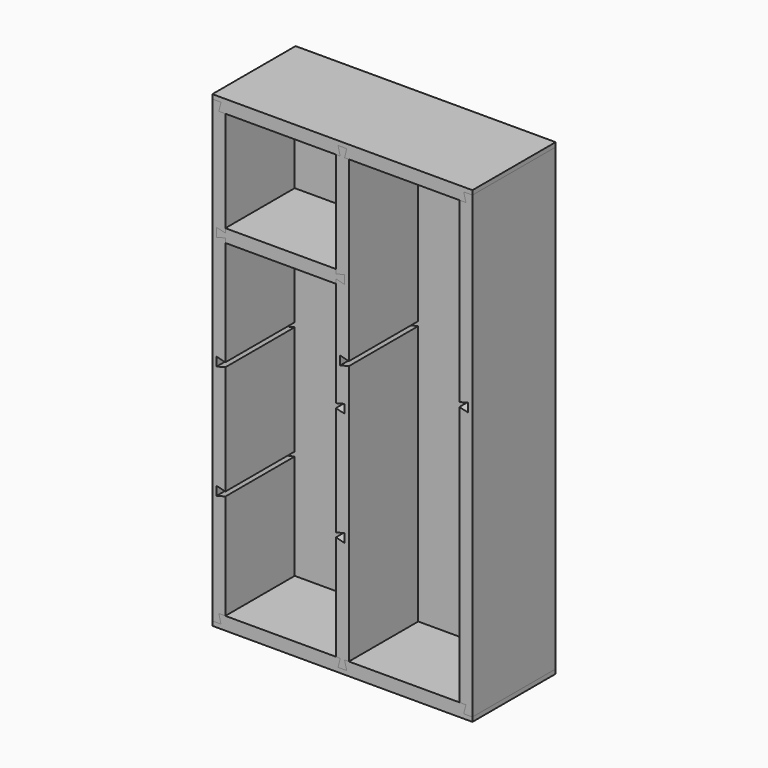
from build123d import *

# Parameters (mm, degrees)
F1_DEPTH  = 152.4
F2_DEPTH  = 152.4
F3_W      = 19.05
F3_H      = 19.05
F4_DEPTH  = 12.7
F6_W      = 361.95
F6_H      = 666.75
F7_DEPTH  = 5.55625
F8_W      = 360.3625
F8_H      = 665.1625
F9_DEPTH  = 4.99999
F11_DEPTH = 127
F13_DEPTH = 127


# Not quite as in the source:
# - a feature names something its author has since deleted; it is built from what else it names


with BuildPart() as f1:
    # F0 (on Front) → F1 (new body)
    with BuildSketch(Plane.XZ):
        Polygon((-180.9664656361, 323.85), (-190.5, 323.85), (-190.5, -323.85), (-180.9664656361, -323.85), (-171.45, -323.85), (-171.45, -176.2125), (-171.45, -169.8710343639), (-184.15, -173.0375), (-184.15, -160.3375), (-171.45, -163.5039656361), (-171.45, -157.1625), (-171.45, -9.525), (-171.45, -3.1835343639), (-184.15, -6.35), (-184.15, 6.35), (-171.45, 3.1835343639), (-171.45, 9.525), (-171.45, 157.1625), (-171.45, 163.5039656361), (-184.15, 160.3375), (-184.15, 173.0375), (-171.45, 169.8710343639), (-171.45, 176.2125), (-171.45, 323.85), align=None)
        Polygon((-177.8, 336.55), (-190.5, 336.55), (-190.5, 323.85), (-180.9664656361, 323.85), align=None)
        Polygon((-180.9664656361, -323.85), (-190.5, -323.85), (-190.5, -336.55), (-177.8, -336.55), align=None)
    extrude(amount=F1_DEPTH)


with BuildPart() as f1b:
    # F0 (on Front) → F1, piece 2 (new body)
    with BuildSketch(Plane.XZ):
        Polygon((190.5, -323.85), (190.5, 323.85), (180.9664656361, 323.85), (171.45, 323.85), (171.45, 69.85), (171.45, 63.5085343639), (184.15, 66.675), (184.15, 53.975), (171.45, 57.1414656361), (171.45, 50.8), (171.45, -323.85), (180.9664656361, -323.85), align=None)
        Polygon((190.5, -336.55), (190.5, -323.85), (180.9664656361, -323.85), (177.8, -336.55), align=None)
        Polygon((190.5, 323.85), (190.5, 336.55), (177.8, 336.55), (180.9664656361, 323.85), align=None)
    extrude(amount=F1_DEPTH)


with BuildPart() as f2:
    # F0 (on Front) → F2 (new body, through all)
    with BuildSketch(Plane.XZ):
        Polygon((190.5, 336.55), (190.5, 342.9), (-190.5, 342.9), (-190.5, 336.55), (-177.8, 336.55), (-180.9664656361, 323.85), (-171.45, 323.85), (-9.525, 323.85), (-3.1835343639, 323.85), (-6.35, 336.55), (6.35, 336.55), (3.1835343639, 323.85), (9.525, 323.85), (171.45, 323.85), (180.9664656361, 323.85), (177.8, 336.55), align=None)
    extrude(amount=F2_DEPTH)


with BuildPart() as f2b:
    # F0 (on Front) → F2, piece 2 (new body, through all)
    with BuildSketch(Plane.XZ):
        Polygon((190.5, -342.9), (190.5, -336.55), (177.8, -336.55), (180.9664656361, -323.85), (171.45, -323.85), (9.525, -323.85), (9.525, -342.9), align=None)
        Polygon((-9.525, -342.9), (9.525, -342.9), (9.525, -323.85), (3.1835343639, -323.85), (6.35, -336.55), (-6.35, -336.55), (-3.1835343639, -323.85), (-9.525, -323.85), align=None)
        Polygon((-177.8, -336.55), (-190.5, -336.55), (-190.5, -342.9), (-9.525, -342.9), (-9.525, -323.85), (-171.45, -323.85), (-180.9664656361, -323.85), align=None)
    extrude(amount=F2_DEPTH)

    # F3 (on face) → F4 (cut)
    with BuildSketch(Plane(origin=(0, 0, 0), x_dir=(-1, 0, 0), z_dir=(0, 1, 0))):
        with Locations((155.575, -333.375)):
            Rectangle(F3_W, F3_H)
    extrude(amount=-F4_DEPTH, mode=Mode.SUBTRACT)


with BuildPart() as f7_tool:
    # F6 (on offset) → F7 (new body)
    with BuildSketch(Plane.XZ.offset(25.4)):
        Rectangle(F6_W, F6_H)
    extrude(amount=-F7_DEPTH)


with BuildPart() as f1_1:
    add(f1.part)

    # F7: cut by f7_tool
    add(f7_tool.part, mode=Mode.SUBTRACT)


with BuildPart() as f1b_1:
    add(f1b.part)

    # F7: cut by f7_tool
    add(f7_tool.part, mode=Mode.SUBTRACT)


with BuildPart() as f2_1:
    add(f2.part)

    # F7: cut by f7_tool
    add(f7_tool.part, mode=Mode.SUBTRACT)


with BuildPart() as f2b_1:
    add(f2b.part)

    # F7: cut by f7_tool
    add(f7_tool.part, mode=Mode.SUBTRACT)


with BuildPart() as f9:
    # F8 (on offset) → F9 (new body)
    with BuildSketch(Plane.XZ.offset(25.4)):
        Rectangle(F8_W, F8_H)
    extrude(amount=-F9_DEPTH)


with BuildPart() as f11:
    # F10 (on face) → F11 (new body, through all)
    with BuildSketch(Plane.XZ.offset(25.4)):
        Polygon((-5.3604794887, 332.58125), (5.3604794887, 332.58125), (6.35, 336.55), (-6.35, 336.55), align=None)
        Polygon((6.35, -336.55), (5.3604794887, -332.58125), (-5.3604794887, -332.58125), (-6.35, -336.55), align=None)
        Polygon((9.525, 63.5085343639), (9.525, 323.85), (3.1835343639, 323.85), (5.3604794887, 332.58125), (-5.3604794887, 332.58125), (-3.1835343639, 323.85), (-9.525, 323.85), (-9.525, 169.8710343639), (3.175, 173.0375), (3.175, 160.3375), (-9.525, 163.5039656361), (-9.525, 3.1835343639), (3.175, 6.35), (3.175, -6.35), (-9.525, -3.1835343639), (-9.525, -163.5039656361), (3.175, -160.3375), (3.175, -173.0375), (-9.525, -169.8710343639), (-9.525, -323.85), (-3.1835343639, -323.85), (-5.3604794887, -332.58125), (5.3604794887, -332.58125), (3.1835343639, -323.85), (9.525, -323.85), (9.525, 57.1414656361), (-3.175, 53.975), (-3.175, 66.675), align=None)
    extrude(amount=F11_DEPTH)


with BuildPart() as f13:
    # F12 (on face) → F13 (new body, through all)
    with BuildSketch(Plane.XZ.offset(25.4)):
        Polygon((-9.525, 169.8710343639), (-9.525, 176.2125), (-171.45, 176.2125), (-171.45, 169.8710343639), (-184.15, 173.0375), (-184.15, 160.3375), (-171.45, 163.5039656361), (-171.45, 157.1625), (-9.525, 157.1625), (-9.525, 163.5039656361), (3.175, 160.3375), (3.175, 173.0375), align=None)
    extrude(amount=F13_DEPTH)


solid = Compound([f1_1.part, f1b_1.part, f2_1.part, f2b_1.part, f9.part, f11.part, f13.part])
